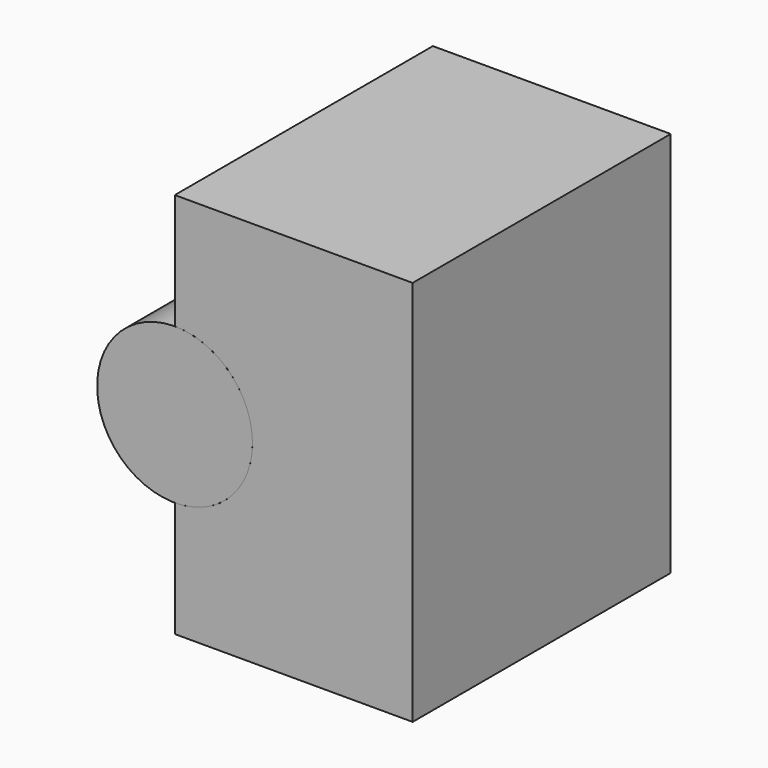
from build123d import *

# Parameters (mm, degrees)
F0_R     = 38.1
F1_DEPTH = 25.4
F3_DEPTH = 158.242
F4_DEPTH = 132.842


with BuildPart() as f1:
    # F0 (on Front) → F1 (new body)
    with BuildSketch(Plane.XZ):
        Circle(F0_R)
    extrude(amount=F1_DEPTH)

    # F4 (add, through all): a face of the model
    f4_faces = [f1.faces().sort_by_distance(p)[0] for p in [
        (0, -25.4, 0),
    ]]
    extrude(f4_faces, amount=F4_DEPTH)


with BuildPart() as f3:
    # F2 (on Front) → F3 (new body)
    with BuildSketch(Plane.XZ):
        with BuildLine():
            ThreePointArc((0, 38.1), (38.1, 0), (0, -38.1))
            Line((0, -38.1), (0, -94.7943329811))
            Line((0, -94.7943329811), (116.6753321886, -94.7943329811))
            Line((116.6753321886, -94.7943329811), (116.6753321886, 0))
            Line((116.6753321886, 0), (116.6753321886, 94.7943329811))
            Line((116.6753321886, 94.7943329811), (0, 94.7943329811))
            Line((0, 94.7943329811), (0, 38.1))
        make_face()
    extrude(amount=F3_DEPTH)


solid = Compound([f1.part, f3.part])
